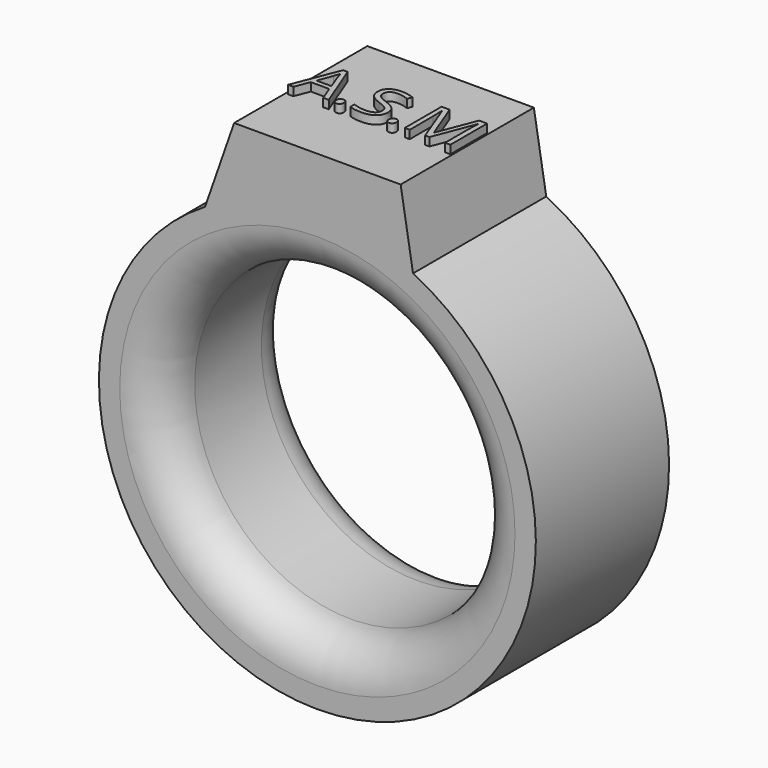
from build123d import *

# Parameters (mm, degrees)
F0_R         = 13.32865
F0_R_2       = 9.51865
F1_DEPTH     = 10.16
F3_DEPTH     = 10.16
F4_R         = 2.54
F5_TEXT_SIZE = 3.9320312028
F6_DEPTH     = 0.508


# Not quite as in the source:
# - Text() gives the source's letters only with a copy of the font that has no kerning and outlines rounded to 1/6400 em; it was checked with that copy


with BuildPart() as f1:
    # F0 (on Front) → F1 (new body)
    with BuildSketch(Plane.XZ):
        with Locations((-2.4824102875, 13.3668258786)):
            Circle(F0_R)
        with Locations((-2.4824102875, 13.3668258786)):
            Circle(F0_R_2, mode=Mode.SUBTRACT)
    extrude(amount=-F1_DEPTH)

    # F2 (on Front) → F3 (join)
    with BuildSketch(Plane.XZ):
        with BuildLine():
            ThreePointArc((-9.335067846, 24.7989733238), (-3.0609255375, 26.682915054), (3.3529637647, 25.3502027188))
            Line((3.3529637647, 25.3502027188), (2.5975897125, 29.8789733238))
            Line((2.5975897125, 29.8789733238), (-7.5624102875, 29.8789733238))
            Line((-7.5624102875, 29.8789733238), (-9.335067846, 24.7989733238))
        make_face()
    extrude(amount=-F3_DEPTH)

    # F4
    f4_edges = [f1.edges().sort_by_distance(p)[0] for p in [
        (-12.00106, 0, 13.366826),
        (-12.00106, 10.16, 13.366826),
    ]]
    fillet(f4_edges, radius=F4_R)

    # F5 (on face) → F6 (join)
    with BuildSketch(Plane.XY.offset(29.8789733238)):
        with Locations((-7.4100102875, 3.918682701)):
            Text('A.S.M', F5_TEXT_SIZE, font='Open Sans', text_align=(TextAlign.LEFT, TextAlign.BOTTOM))
    extrude(amount=F6_DEPTH)


solid = f1.part
